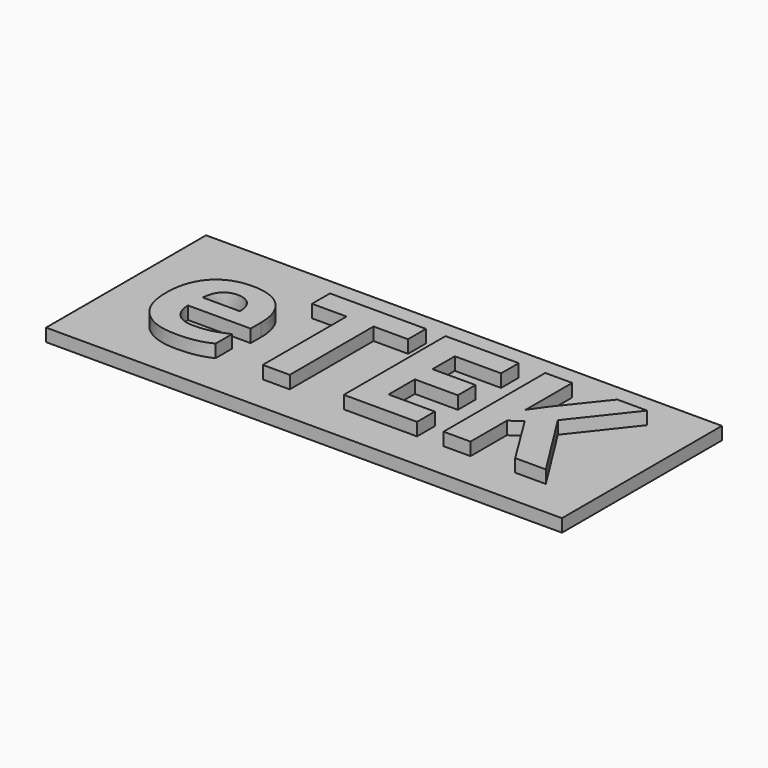
from build123d import *

# Parameters (mm, degrees)
F0_TEXT_SIZE = 13.8888888889
F1_DEPTH     = 1
F0_W         = 40.2328602504
F0_H         = 15.5926402658
F2_DEPTH     = 1
F3_DEPTH     = 1


# Not quite as in the source:
# - Text() gives the source's letters only with a copy of the font that has no kerning and outlines rounded to 1/6400 em; it was checked with that copy


with BuildPart() as f1:
    # F0 (on Top) → F1 (new body)
    with BuildSketch(Plane.XY):
        with Locations((0, -10)):
            Text('eTEK', F0_TEXT_SIZE, font='Open Sans', font_style=FontStyle.BOLD, text_align=(TextAlign.LEFT, TextAlign.BOTTOM))
    extrude(amount=F1_DEPTH)


with BuildPart() as f2:
    # F0 (on Top) → F2 (new body)
    with BuildSketch(Plane.XY):
        with Locations((16.7161297286, -5.1087737083)):
            Rectangle(F0_W, F0_H)
        with BuildLine():
            add(Edge.make_bspline(
                [(6.0221354167, -10.0043402778), (5.4058159722, -10.13671875), (4.5160590278, -10.13671875)],
                knots=[0, 0, 0, 1, 1, 1], degree=2))
            add(Edge.make_bspline(
                [(4.5160590278, -10.13671875), (2.6866319444, -10.13671875), (1.6558159722, -9.1254340278)],
                knots=[0, 0, 0, 1, 1, 1], degree=2))
            add(Edge.make_bspline(
                [(1.6558159722, -9.1254340278), (0.625, -8.1141493056), (0.625, -6.2630208333)],
                knots=[0, 0, 0, 1, 1, 1], degree=2))
            add(Edge.make_bspline(
                [(0.625, -6.2630208333), (0.625, -4.3576388889), (1.5776909722, -3.3170572917)],
                knots=[0, 0, 0, 1, 1, 1], degree=2))
            add(Edge.make_bspline(
                [(1.5776909722, -3.3170572917), (2.5303819444, -2.2764756944), (4.2122395833, -2.2764756944)],
                knots=[0, 0, 0, 1, 1, 1], degree=2))
            add(Edge.make_bspline(
                [(4.2122395833, -2.2764756944), (5.8181423611, -2.2764756944), (6.7133246528, -3.1911892361)],
                knots=[0, 0, 0, 1, 1, 1], degree=2))
            add(Edge.make_bspline(
                [(6.7133246528, -3.1911892361), (7.6085069444, -4.1059027778), (7.6085069444, -5.7204861111)],
                knots=[0, 0, 0, 1, 1, 1], degree=2))
            Line((7.6085069444, -5.7204861111), (7.6085069444, -6.7252604167))
            Line((7.6085069444, -6.7252604167), (2.7191840278, -6.7252604167))
            add(Edge.make_bspline(
                [(2.7191840278, -6.7252604167), (2.75390625, -7.6063368056), (3.2421875, -8.1011284722)],
                knots=[0, 0, 0, 1, 1, 1], degree=2))
            add(Edge.make_bspline(
                [(3.2421875, -8.1011284722), (3.73046875, -8.5959201389), (4.6115451389, -8.5959201389)],
                knots=[0, 0, 0, 1, 1, 1], degree=2))
            add(Edge.make_bspline(
                [(4.6115451389, -8.5959201389), (5.2973090278, -8.5959201389), (5.9071180556, -8.4537760417)],
                knots=[0, 0, 0, 1, 1, 1], degree=2))
            add(Edge.make_bspline(
                [(5.9071180556, -8.4537760417), (6.5169270833, -8.3116319444), (7.1809895833, -7.9991319444)],
                knots=[0, 0, 0, 1, 1, 1], degree=2))
            Line((7.1809895833, -7.9991319444), (7.1809895833, -9.6006944444))
            add(Edge.make_bspline(
                [(7.1809895833, -9.6006944444), (6.6384548611, -9.8719618056), (6.0221354167, -10.0043402778)],
                knots=[0, 0, 0, 1, 1, 1], degree=2))
        make_face(mode=Mode.SUBTRACT)
        Polygon((13.2790798611, -1.8337673611), (13.2790798611, -10), (11.1762152778, -10), (11.1762152778, -1.8337673611), (8.4830729167, -1.8337673611), (8.4830729167, -0.0846354167), (15.9700520833, -0.0846354167), (15.9700520833, -1.8337673611), align=None, mode=Mode.SUBTRACT)
        Polygon((23.2052951389, -8.2638888889), (23.2052951389, -10), (17.4956597222, -10), (17.4956597222, -0.0846354167), (23.2052951389, -0.0846354167), (23.2052951389, -1.8077256944), (19.5985243056, -1.8077256944), (19.5985243056, -3.984375), (22.9557291667, -3.984375), (22.9557291667, -5.7074652778), (19.5985243056, -5.7074652778), (19.5985243056, -8.2638888889), align=None, mode=Mode.SUBTRACT)
        Polygon((29.7634548611, -4.47265625), (33.2486979167, -10), (30.8615451389, -10), (28.2638888889, -5.8224826389), (27.3763020833, -6.4605034722), (27.3763020833, -10), (25.2734375, -10), (25.2734375, -0.0846354167), (27.3763020833, -0.0846354167), (27.3763020833, -4.6223958333), (28.203125, -3.4548611111), (30.8897569444, -0.0846354167), (33.22265625, -0.0846354167), align=None, mode=Mode.SUBTRACT)
    extrude(amount=-F2_DEPTH)


with BuildPart() as f3:
    # F0 (on Top) → F3 (new body)
    with BuildSketch(Plane.XY):
        with Locations((0, -10)):
            Text('eTEK', F0_TEXT_SIZE, font='Open Sans', font_style=FontStyle.BOLD, text_align=(TextAlign.LEFT, TextAlign.BOTTOM))
    extrude(amount=-F3_DEPTH)


solid = Compound([f1.part, f2.part, f3.part])
